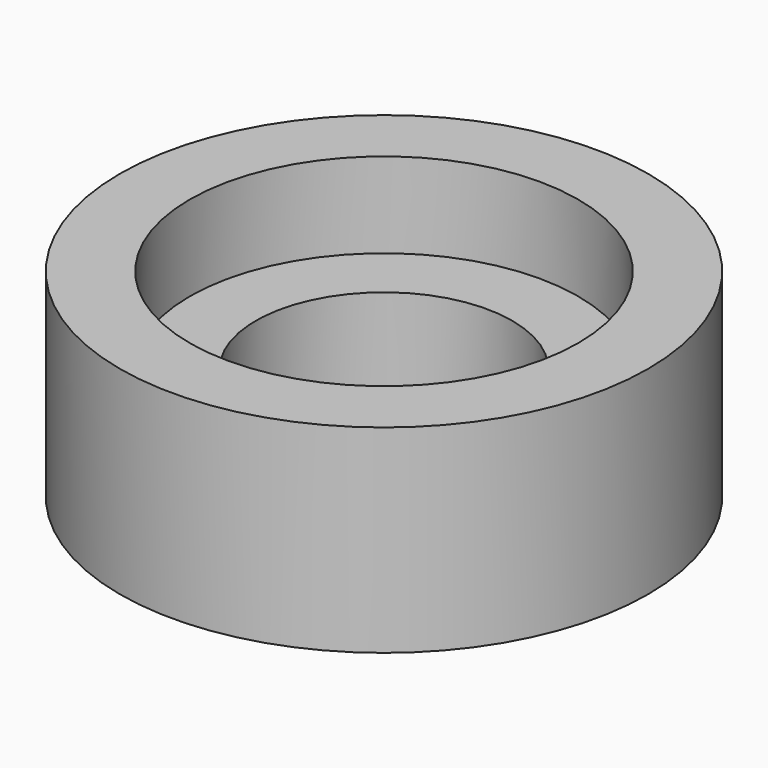
from build123d import *

# Parameters (mm, degrees)
F0_R     = 5.15
F0_R_2   = 3.4
F1_DEPTH = 3
F0_R_3   = 7
F2_DEPTH = 5.26


# Not quite as in the source:
# - a feature names something its author has since deleted; it is built from what else it names


with BuildPart() as f1:
    # F0 (on Top) → F1 (new body)
    with BuildSketch(Plane.XY):
        Circle(F0_R)
        Circle(F0_R_2, mode=Mode.SUBTRACT)
    extrude(amount=F1_DEPTH)

    # F0 (on Top) → F2 (join)
    with BuildSketch(Plane.XY):
        Circle(F0_R_3)
        Circle(F0_R, mode=Mode.SUBTRACT)
    extrude(amount=F2_DEPTH)


solid = f1.part
